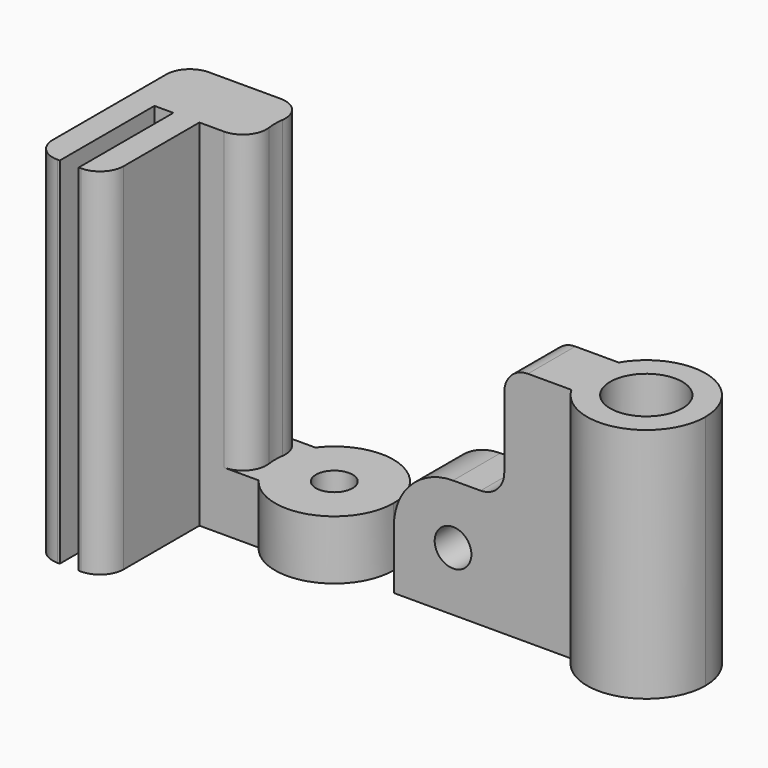
from build123d import *

# Parameters (mm, degrees)
F0_R      = 1.55
F1_DEPTH  = 5
F2_DEPTH  = 30
F3_R      = 2
F4_R      = 3.05
F5_DEPTH  = 20
F6_DEPTH  = 10
F7_R      = 1.55
F8_DEPTH  = 25
F10_DEPTH = 10
F11_R     = 0.9
F12_DEPTH = 10
F13_R     = 2


with BuildPart() as f1:
    # F0 (on Top) → F1 (new body)
    with BuildSketch(Plane.XY):
        with BuildLine():
            ThreePointArc((-4, -3), (1.5811388301, -4.7434164903), (5, 0))
            ThreePointArc((5, 0), (1.5811388301, 4.7434164903), (-4, 3))
            ThreePointArc((-4, 3), (-5, 0), (-4, -3))
        make_face()
        Circle(F0_R, mode=Mode.SUBTRACT)
    extrude(amount=F1_DEPTH)

    # F0 (on Top) → F2 (join)
    with BuildSketch(Plane.XY):
        with BuildLine():
            ThreePointArc((-4, -3), (-5, 0), (-4, 3))
            Line((-4, 3), (-15, 3))
            Line((-15, 3), (-15, -13))
            Line((-15, -13), (-12.8, -13))
            Line((-12.8, -13), (-12.8, -3))
            Line((-12.8, -3), (-11.2, -3))
            Line((-11.2, -3), (-11.2, -13))
            Line((-11.2, -13), (-9, -13))
            Line((-9, -13), (-9, -3))
            Line((-9, -3), (-4, -3))
        make_face()
    extrude(amount=F2_DEPTH)

    # F3
    f3_edges = [f1.edges().sort_by_distance(p)[0] for p in [
        (-4, 3, 17.5),
        (-4, -3, 17.5),
        (-15, 3, 15),
        (-9, -13, 15),
        (-15, -13, 15),
    ]]
    fillet(f3_edges, radius=F3_R)


with BuildPart() as f5:
    # F4 (on Top) → F5 (new body)
    with BuildSketch(Plane.XY):
        with BuildLine():
            ThreePointArc((22.0380171016, -2.5), (27.662239346, -4.8296291314), (31.3681441205, 0))
            ThreePointArc((31.3681441205, 0), (27.662239346, 4.8296291314), (22.0380171016, 2.5))
            ThreePointArc((22.0380171016, 2.5), (21.3681441205, 0), (22.0380171016, -2.5))
        make_face()
        with Locations((26.3681441205, 0)):
            Circle(F4_R, mode=Mode.SUBTRACT)
    extrude(amount=F5_DEPTH)

    # F4 (on Top) → F6 (join)
    with BuildSketch(Plane.XY):
        with BuildLine():
            ThreePointArc((22.0380171016, -2.5), (21.3681441205, 0), (22.0380171016, 2.5))
            Line((22.0380171016, 2.5), (7.0380171016, 2.5))
            Line((7.0380171016, 2.5), (7.0380171016, -2.5))
            Line((7.0380171016, -2.5), (22.0380171016, -2.5))
        make_face()
    extrude(amount=F6_DEPTH)

    # F7 (on face) → F8 (cut)
    with BuildSketch(Plane.XZ.offset(2.5)):
        with BuildLine():
            ThreePointArc((7.0380171016, 5), (8.5024831957, 8.5355339059), (12.0380171016, 10))
            Line((12.0380171016, 10), (7.0380171016, 10))
            Line((7.0380171016, 10), (7.0380171016, 5))
        make_face()
        with Locations((12.0380171016, 5)):
            Circle(F7_R)
    extrude(amount=-F8_DEPTH, mode=Mode.SUBTRACT)

    # F9 (on face) → F10 (join)
    with BuildSketch(Plane.XY.offset(10)):
        with BuildLine():
            Line((22.0380171016, 2.5), (16.3681441205, 2.5))
            Line((16.3681441205, 2.5), (16.3681441205, -2.5))
            Line((16.3681441205, -2.5), (22.0380171016, -2.5))
            ThreePointArc((22.0380171016, -2.5), (21.3681441205, 0), (22.0380171016, 2.5))
        make_face()
    extrude(amount=F10_DEPTH)

    # F11 (on face) → F12 (cut)
    with BuildSketch(Plane(origin=(16.3681441205, 0, 0), x_dir=(0, -1, 0), z_dir=(-1, 0, 0))):
        with Locations((0, 15)):
            Circle(F11_R)
    extrude(amount=-F12_DEPTH, mode=Mode.SUBTRACT)

    # F13
    f13_edges = [f5.edges().sort_by_distance(p)[0] for p in [
        (16.368144, 0, 20),
        (16.368144, 0, 10),
    ]]
    fillet(f13_edges, radius=F13_R)


solid = Compound([f1.part, f5.part])
